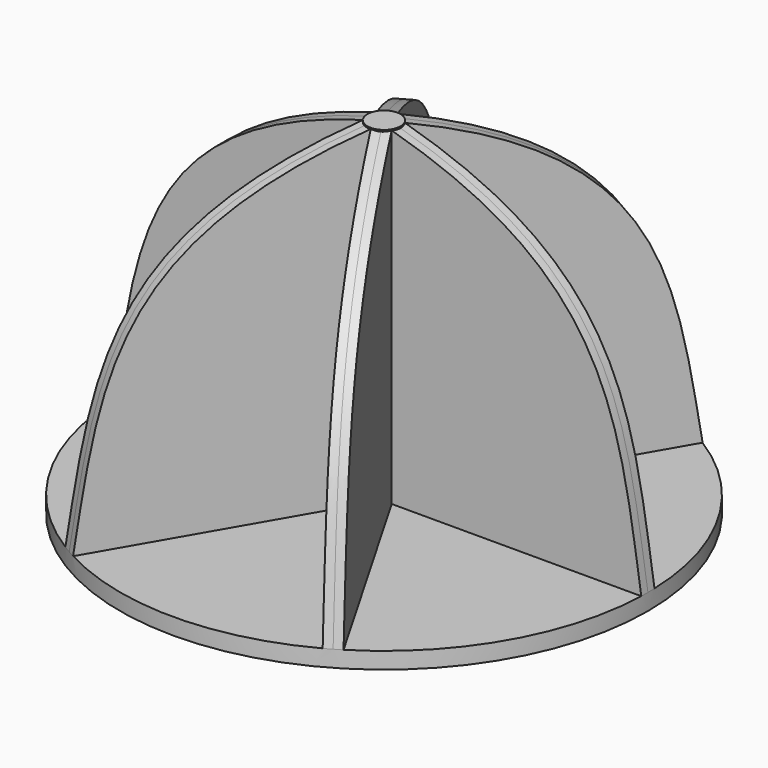
from build123d import *

# Parameters (mm, degrees)
F0_R            = 25.4
F1_DEPTH        = 1.5875
F2_R            = 1.5875
F3_DEPTH        = 31.75
F5_DEPTH        = 0.79375
F5_COPIES_COUNT = 6


# Not quite as in the source:
# - a pattern or mirror of a feature is missing from the dataset's text; its kind, count and spacing are read off the source's solid


with BuildPart() as f1:
    # F0 (on Top) → F1 (new body)
    with BuildSketch(Plane.XY):
        Circle(F0_R)
    extrude(amount=F1_DEPTH)

    # F2 (on face) → F3 (join)
    with BuildSketch(Plane.XY.offset(1.5875)):
        Circle(F2_R)
    extrude(amount=F3_DEPTH)

    # F4 (on Front) → F5 (join, symmetric)
    with BuildSketch(Plane.XZ):
        with BuildLine():
            Line((1.016, 33.3375), (1.016, 1.5875))
            Line((1.016, 1.5875), (25.4, 1.5875))
            add(Edge.make_bspline(
                [(1.016, 33.3375), (22.407008335, 27.4323299527), (23.2129693031, 15.8802140504), (25.4, 1.5875)],
                knots=[0, 0, 0, 0, 40.0330108286, 40.0330108286, 40.0330108286, 40.0330108286], degree=3))
        make_face()
    f5 = extrude(amount=F5_DEPTH, both=True)

    # F5_copies: F5 ×6 about axis
    f5_copies_axis = Axis((0, 0, 0), (0, 0, 1))
    for i in range(1, F5_COPIES_COUNT):
        add(f5.rotate(f5_copies_axis, i * 360 / F5_COPIES_COUNT))


solid = f1.part
